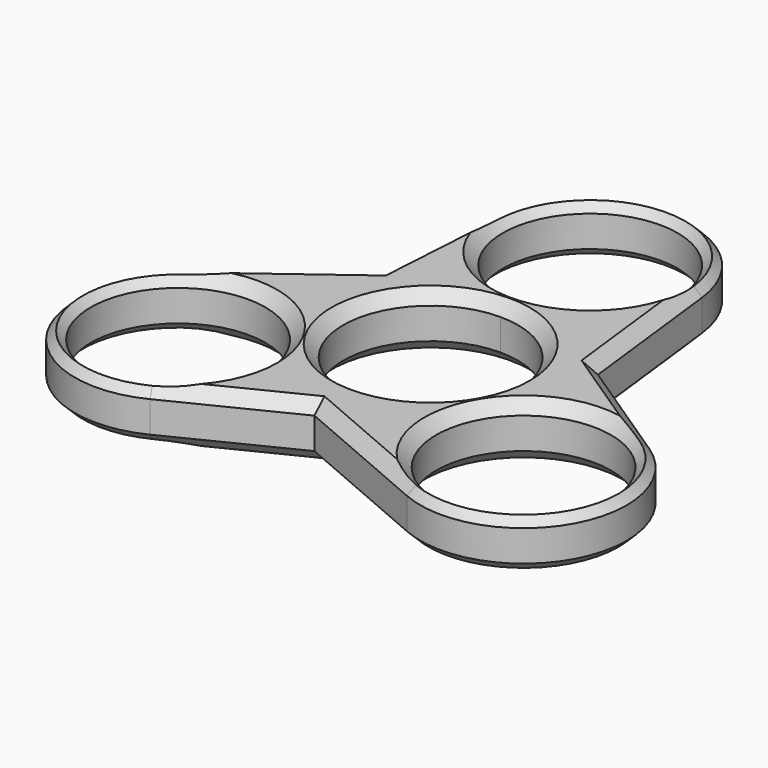
from build123d import *

# Parameters (mm, degrees)
F0_R         = 11.2
F1_DEPTH     = 7
F2_T4_DEPTH  = 23.5617897445
F2_T7_ANGLE  = 169.7193644143
F2_T11_DEPTH = 20.6774904565
F2_T16_DEPTH = 23.5617897445
F2_T19_ANGLE = 169.7193644143
F2_T23_DEPTH = 20.6774904565
F2_T28_DEPTH = 23.5617897445
F2_T31_ANGLE = 169.7193644143
F2_T35_DEPTH = 20.6774904565
F2_T49_DEPTH = 23.5617897445
F2_T53_DEPTH = 20.6774904565
F2_T60_DEPTH = 20.6774904565
F2_T64_DEPTH = 23.5617897445
F2_T71_DEPTH = 20.6774904565
F2_T75_DEPTH = 23.5617897445
F3_T4_DEPTH  = 23.5617897445
F3_T7_ANGLE  = 169.7193644143
F3_T11_DEPTH = 20.6774904565
F3_T16_DEPTH = 23.5617897445
F3_T19_ANGLE = 169.7193644143
F3_T23_DEPTH = 20.6774904565
F3_T28_DEPTH = 23.5617897445
F3_T31_ANGLE = 169.7193644143
F3_T35_DEPTH = 20.6774904565
F3_T49_DEPTH = 23.5617897445
F3_T53_DEPTH = 20.6774904565
F3_T60_DEPTH = 23.5617897445
F3_T64_DEPTH = 20.6774904565
F3_T71_DEPTH = 23.5617897445
F3_T75_DEPTH = 20.6774904565


# Not quite as in the source:
# - a fillet or chamfer that OpenCascade refuses, or shapes differently, is made with other operations: its cross-section is extruded or revolved along the edge and cut away or added


with BuildPart() as f1:
    # F0 (on Top) → F1 (new body)
    with BuildSketch(Plane.XY):
        with BuildLine():
            Line((15.4120276741, 7.5237850523), (13.109573538, 27.0930664517))
            ThreePointArc((13.109573538, 27.0930664517), (-0.3616695295, 38.7456835975), (-13.1743812219, 26.3726364702))
            Line((-13.1743812219, 26.3726364702), (-14.221802825, 9.5853149634))
            Line((-14.221802825, 9.5853149634), (-30.0180705826, -2.1933095092))
            ThreePointArc((-30.0180705826, -2.1933095092), (-33.3739115177, -19.686056799), (-16.252182537, -24.5956670524))
            Line((-16.252182537, -24.5956670524), (-1.1902248491, -17.1091000158))
            Line((-1.1902248491, -17.1091000158), (16.9084970446, -24.8997569426))
            ThreePointArc((16.9084970446, -24.8997569426), (33.7355810471, -19.0596267984), (29.4265637589, -1.7769694177))
            Line((29.4265637589, -1.7769694177), (15.4120276741, 7.5237850523))
        make_face()
        with Locations((-22.1275026794, -12.7753196284)):
            Circle(F0_R, mode=Mode.SUBTRACT)
        with Locations((22.1275026794, -12.7753196284)):
            Circle(F0_R, mode=Mode.SUBTRACT)
        with BuildLine():
            ThreePointArc((0, 11.2), (7.9195959493, 7.9195959493), (11.2, 0))
            ThreePointArc((11.2, 0), (5.6, -9.6994845224), (-5.6, -9.6994845224))
            ThreePointArc((-5.6, -9.6994845224), (-10.8183692544, 2.8987733051), (0, 11.2))
        make_face(mode=Mode.SUBTRACT)
        with Locations((0, 25.5506392568)):
            Circle(F0_R, mode=Mode.SUBTRACT)
    extrude(amount=F1_DEPTH)

    # F2: chamfer of 1.5 on 13 edges, made by hand


with BuildPart() as f2_tool2:
    # F2_s3 → F2_t4 (new body)
    with BuildSketch(Plane(origin=(-0.211945286, 1.8013896037, 0), x_dir=(0, 0, 1), z_dir=(-0.1168505451, 0.9931495105, 0))):
        Polygon((5.5, 16.185606124), (7, 14.685606124), (7, 16.185606124), align=None)
    extrude(amount=F2_T4_DEPTH)

    split(bisect_by=Plane(origin=(8.1788758548, 12.3240701783, 0), x_dir=(0, 0, 1), z_dir=(0.5529591727, 0.8332083493, 0)), keep=Keep.TOP)


with BuildPart() as f1_1:
    add(f1.part)

    # F2_t1: cut F2_tool2
    add(f2_tool2.part, mode=Mode.SUBTRACT)

    # F2_s6 → F2_t7 (revolve, cut)
    with BuildSketch(Plane(origin=(-2.9651532605, 25.2017695539, 0), x_dir=(0, 0, 1), z_dir=(0.1168505451, -0.9931495105, 0))):
        Polygon((7, -14.685606124), (5.5, -16.185606124), (7, -16.185606124), align=None)
    revolve(axis=Axis((0, 25.5506392568, 7), (0, 0, 1)), revolution_arc=F2_T7_ANGLE, mode=Mode.SUBTRACT)


with BuildPart() as f2_tool9:
    # F2_s10 → F2_t11 (new body)
    with BuildSketch(Plane(origin=(1.5880145579, 25.4515572947, 0), x_dir=(0, 0, 1), z_dir=(-0.0622725162, -0.9980591835, 0))):
        Polygon((7, 13.2911025961), (5.5, 14.7911025961), (7, 14.7911025961), align=None)
    extrude(amount=F2_T11_DEPTH)

    split(bisect_by=Plane(origin=(-9.6752745589, 12.9754733174, 0), x_dir=(0, 0, 1), z_dir=(-0.5977702957, 0.8016674333, 0)), keep=Keep.TOP)


with BuildPart() as f1_2:
    add(f1_1.part)

    # F2_t8: cut F2_tool9
    add(f2_tool9.part, mode=Mode.SUBTRACT)


with BuildPart() as f2_tool14:
    # F2_s15 → F2_t16 (new body)
    with BuildSketch(Plane(origin=(-1.4540765159, -1.0842448037, 0), x_dir=(0, 0, 1), z_dir=(-0.8016674333, -0.5977702957, 0))):
        Polygon((7, 14.685606124), (5.5, 16.185606124), (7, 16.185606124), align=None)
    extrude(amount=F2_T16_DEPTH)

    split(bisect_by=Plane(origin=(-14.7623957799, 0.9210791755, 0), x_dir=(0, 0, 1), z_dir=(-0.9980591835, 0.0622725162, 0)), keep=Keep.TOP)


with BuildPart() as f1_3:
    add(f1_2.part)

    # F2_t13: cut F2_tool14
    add(f2_tool14.part, mode=Mode.SUBTRACT)

    # F2_s18 → F2_t19 (revolve, cut)
    with BuildSketch(Plane(origin=(-20.3427960238, -15.1687828266, 0), x_dir=(0, 0, 1), z_dir=(0.8016674333, 0.5977702957, 0))):
        Polygon((7, -14.685606124), (5.5, -16.185606124), (7, -16.185606124), align=None)
    revolve(axis=Axis((-22.1275026794, -12.7753196284, 7), (0, 0, 1)), revolution_arc=F2_T19_ANGLE, mode=Mode.SUBTRACT)


with BuildPart() as f2_tool21:
    # F2_s22 → F2_t23 (new body)
    with BuildSketch(Plane(origin=(-22.835702462, -11.3505176986, 0), x_dir=(0, 0, 1), z_dir=(0.8954808655, 0.4451000108, 0))):
        Polygon((7, 13.2911025961), (5.5, 14.7911025961), (7, 14.7911025961), align=None)
    extrude(amount=F2_T23_DEPTH)

    split(bisect_by=Plane(origin=(-6.3994522396, -14.8667702153, 0), x_dir=(0, 0, 1), z_dir=(-0.3953792148, -0.9185179783, 0)), keep=Keep.TOP)


with BuildPart() as f1_4:
    add(f1_3.part)

    # F2_t20: cut F2_tool21
    add(f2_tool21.part, mode=Mode.SUBTRACT)


with BuildPart() as f2_tool26:
    # F2_s27 → F2_t28 (new body)
    with BuildSketch(Plane(origin=(1.6660218019, -0.7171447999, 0), x_dir=(0, 0, 1), z_dir=(0.9185179783, -0.3953792148, 0))):
        Polygon((7, 14.685606124), (5.5, 16.185606124), (7, 16.185606124), align=None)
    extrude(amount=F2_T28_DEPTH)

    split(bisect_by=Plane(origin=(6.5835199251, -13.2451493538, 0), x_dir=(0, 0, 1), z_dir=(0.4451000108, -0.8954808655, 0)), keep=Keep.TOP)


with BuildPart() as f1_5:
    add(f1_4.part)

    # F2_t25: cut F2_tool26
    add(f2_tool26.part, mode=Mode.SUBTRACT)

    # F2_s30 → F2_t31 (revolve, cut)
    with BuildSketch(Plane(origin=(23.3079492842, -10.0329867273, 0), x_dir=(0, 0, 1), z_dir=(-0.9185179783, 0.3953792148, 0))):
        Polygon((7, -14.685606124), (5.5, -16.185606124), (7, -16.185606124), align=None)
    revolve(axis=Axis((22.1275026794, -12.7753196284, 7), (0, 0, 1)), revolution_arc=F2_T31_ANGLE, mode=Mode.SUBTRACT)


with BuildPart() as f2_tool33:
    # F2_s34 → F2_t35 (new body)
    with BuildSketch(Plane(origin=(21.2476879041, -14.1010395961, 0), x_dir=(0, 0, 1), z_dir=(-0.8332083493, 0.5529591727, 0))):
        Polygon((7, 13.2911025961), (5.5, 14.7911025961), (7, 14.7911025961), align=None)
    extrude(amount=F2_T35_DEPTH)

    split(bisect_by=Plane(origin=(16.0747267985, 1.8912968978, 0), x_dir=(0, 0, 1), z_dir=(0.9931495105, 0.1168505451, 0)), keep=Keep.TOP)


with BuildPart() as f1_6:
    add(f1_5.part)

    # F2_t32: cut F2_tool33
    add(f2_tool33.part, mode=Mode.SUBTRACT)

    # F2_s37 → F2_t38 (revolve, cut)
    with BuildSketch(Plane.XZ.offset(12.7753196284)):
        Polygon((-9.4275026794, 7), (-10.9275026794, 5.5), (-10.9275026794, 7), align=None)
    revolve(axis=Axis((-22.1275026794, -12.7753196284, 7), (0, 0, 1)), mode=Mode.SUBTRACT)

    # F2_s39 → F2_t40 (revolve, cut)
    with BuildSketch(Plane.XZ.offset(12.7753196284)):
        Polygon((34.8275026794, 7), (33.3275026794, 5.5), (33.3275026794, 7), align=None)
    revolve(axis=Axis((22.1275026794, -12.7753196284, 7), (0, 0, 1)), mode=Mode.SUBTRACT)

    # F2_s41 → F2_t42 (revolve, cut)
    with BuildSketch(Plane(origin=(0, 0, 0), x_dir=(0, 0, 1), z_dir=(-0.8660254038, 0.5, 0))):
        Polygon((7, -12.7), (5.5, -11.2), (7, -11.2), align=None)
    revolve(axis=Axis((0, 0, 7), (0, 0, 1)), mode=Mode.SUBTRACT)

    # F2_s43 → F2_t44 (revolve, cut)
    with BuildSketch(Plane.XZ.offset(-25.5506392568)):
        Polygon((12.7, 7), (11.2, 5.5), (11.2, 7), align=None)
    revolve(axis=Axis((0, 25.5506392568, 7), (0, 0, 1)), mode=Mode.SUBTRACT)


with BuildPart() as f2_tool47:
    # F2_s48 → F2_t49 (new body)
    with BuildSketch(Plane(origin=(-0.211945286, 1.8013896037, 0), x_dir=(0, 0, 1), z_dir=(-0.1168505451, 0.9931495105, 0))):
        Polygon((5.5, 16.185606124), (7, 14.685606124), (7, 16.185606124), align=None)
    extrude(amount=F2_T49_DEPTH)

    split(bisect_by=Plane(origin=(8.1788758548, 12.3240701783, 0), x_dir=(0, 0, 1), z_dir=(-0.5529591727, -0.8332083493, 0)), keep=Keep.TOP)


with BuildPart() as f2_tool51:
    # F2_s52 → F2_t53 (new body)
    with BuildSketch(Plane(origin=(21.2476879041, -14.1010395961, 0), x_dir=(0, 0, 1), z_dir=(-0.8332083493, 0.5529591727, 0))):
        Polygon((7, 13.2911025961), (5.5, 14.7911025961), (7, 14.7911025961), align=None)
    extrude(amount=F2_T53_DEPTH)

    split(bisect_by=Plane(origin=(16.0747267985, 1.8912968978, 0), x_dir=(0, 0, 1), z_dir=(-0.9931495105, -0.1168505451, 0)), keep=Keep.TOP)


with BuildPart() as f2_tool47_1:
    add(f2_tool47.part)

    # F2_t55: intersect F2_tool51
    add(f2_tool51.part, mode=Mode.INTERSECT)


with BuildPart() as f1_7:
    add(f1_6.part)

    # F2_t45: cut F2_tool47
    add(f2_tool47_1.part, mode=Mode.SUBTRACT)


with BuildPart() as f2_tool58:
    # F2_s59 → F2_t60 (new body)
    with BuildSketch(Plane(origin=(1.5880145579, 25.4515572947, 0), x_dir=(0, 0, 1), z_dir=(-0.0622725162, -0.9980591835, 0))):
        Polygon((7, 13.2911025961), (5.5, 14.7911025961), (7, 14.7911025961), align=None)
    extrude(amount=F2_T60_DEPTH)

    split(bisect_by=Plane(origin=(-9.6752745589, 12.9754733174, 0), x_dir=(0, 0, 1), z_dir=(0.5977702957, -0.8016674333, 0)), keep=Keep.TOP)


with BuildPart() as f2_tool62:
    # F2_s63 → F2_t64 (new body)
    with BuildSketch(Plane(origin=(-1.4540765159, -1.0842448037, 0), x_dir=(0, 0, 1), z_dir=(-0.8016674333, -0.5977702957, 0))):
        Polygon((7, 14.685606124), (5.5, 16.185606124), (7, 16.185606124), align=None)
    extrude(amount=F2_T64_DEPTH)

    split(bisect_by=Plane(origin=(-14.7623957799, 0.9210791755, 0), x_dir=(0, 0, 1), z_dir=(0.9980591835, -0.0622725162, 0)), keep=Keep.TOP)


with BuildPart() as f2_tool58_1:
    add(f2_tool58.part)

    # F2_t66: intersect F2_tool62
    add(f2_tool62.part, mode=Mode.INTERSECT)


with BuildPart() as f1_8:
    add(f1_7.part)

    # F2_t56: cut F2_tool58
    add(f2_tool58_1.part, mode=Mode.SUBTRACT)


with BuildPart() as f2_tool69:
    # F2_s70 → F2_t71 (new body)
    with BuildSketch(Plane(origin=(-22.835702462, -11.3505176986, 0), x_dir=(0, 0, 1), z_dir=(0.8954808655, 0.4451000108, 0))):
        Polygon((7, 13.2911025961), (5.5, 14.7911025961), (7, 14.7911025961), align=None)
    extrude(amount=F2_T71_DEPTH)

    split(bisect_by=Plane(origin=(-6.3994522396, -14.8667702153, 0), x_dir=(0, 0, 1), z_dir=(0.3953792148, 0.9185179783, 0)), keep=Keep.TOP)


with BuildPart() as f2_tool73:
    # F2_s74 → F2_t75 (new body)
    with BuildSketch(Plane(origin=(1.6660218019, -0.7171447999, 0), x_dir=(0, 0, 1), z_dir=(0.9185179783, -0.3953792148, 0))):
        Polygon((7, 14.685606124), (5.5, 16.185606124), (7, 16.185606124), align=None)
    extrude(amount=F2_T75_DEPTH)

    split(bisect_by=Plane(origin=(6.5835199251, -13.2451493538, 0), x_dir=(0, 0, 1), z_dir=(-0.4451000108, 0.8954808655, 0)), keep=Keep.TOP)


with BuildPart() as f2_tool69_1:
    add(f2_tool69.part)

    # F2_t77: intersect F2_tool73
    add(f2_tool73.part, mode=Mode.INTERSECT)


with BuildPart() as f1_9:
    add(f1_8.part)

    # F2_t67: cut F2_tool69
    add(f2_tool69_1.part, mode=Mode.SUBTRACT)

    # F3: chamfer of 1.5 on 13 edges, made by hand


with BuildPart() as f3_tool2:
    # F3_s3 → F3_t4 (new body)
    with BuildSketch(Plane(origin=(-0.211945286, 1.8013896037, 0), x_dir=(0, 0, 1), z_dir=(-0.1168505451, 0.9931495105, 0))):
        Polygon((1.5, 16.185606124), (0, 14.685606124), (0, 16.185606124), align=None)
    extrude(amount=F3_T4_DEPTH)

    split(bisect_by=Plane(origin=(8.1788758548, 12.3240701783, 0), x_dir=(0, 0, 1), z_dir=(0.5529591727, 0.8332083493, 0)), keep=Keep.TOP)


with BuildPart() as f1_10:
    add(f1_9.part)

    # F3_t1: cut F3_tool2
    add(f3_tool2.part, mode=Mode.SUBTRACT)

    # F3_s6 → F3_t7 (revolve, cut)
    with BuildSketch(Plane(origin=(-2.9651532605, 25.2017695539, 0), x_dir=(0, 0, 1), z_dir=(0.1168505451, -0.9931495105, 0))):
        Polygon((1.5, -16.185606124), (0, -14.685606124), (0, -16.185606124), align=None)
    revolve(axis=Axis((0, 25.5506392568, 0), (0, 0, 1)), revolution_arc=F3_T7_ANGLE, mode=Mode.SUBTRACT)


with BuildPart() as f3_tool9:
    # F3_s10 → F3_t11 (new body)
    with BuildSketch(Plane(origin=(1.5880145579, 25.4515572947, 0), x_dir=(0, 0, 1), z_dir=(-0.0622725162, -0.9980591835, 0))):
        Polygon((1.5, 14.7911025961), (0, 13.2911025961), (0, 14.7911025961), align=None)
    extrude(amount=F3_T11_DEPTH)

    split(bisect_by=Plane(origin=(-9.6752745589, 12.9754733174, 0), x_dir=(0, 0, 1), z_dir=(-0.5977702957, 0.8016674333, 0)), keep=Keep.TOP)


with BuildPart() as f1_11:
    add(f1_10.part)

    # F3_t8: cut F3_tool9
    add(f3_tool9.part, mode=Mode.SUBTRACT)


with BuildPart() as f3_tool14:
    # F3_s15 → F3_t16 (new body)
    with BuildSketch(Plane(origin=(-1.4540765159, -1.0842448037, 0), x_dir=(0, 0, 1), z_dir=(-0.8016674333, -0.5977702957, 0))):
        Polygon((1.5, 16.185606124), (0, 14.685606124), (0, 16.185606124), align=None)
    extrude(amount=F3_T16_DEPTH)

    split(bisect_by=Plane(origin=(-14.7623957799, 0.9210791755, 0), x_dir=(0, 0, 1), z_dir=(-0.9980591835, 0.0622725162, 0)), keep=Keep.TOP)


with BuildPart() as f1_12:
    add(f1_11.part)

    # F3_t13: cut F3_tool14
    add(f3_tool14.part, mode=Mode.SUBTRACT)

    # F3_s18 → F3_t19 (revolve, cut)
    with BuildSketch(Plane(origin=(-20.3427960238, -15.1687828266, 0), x_dir=(0, 0, 1), z_dir=(0.8016674333, 0.5977702957, 0))):
        Polygon((1.5, -16.185606124), (0, -14.685606124), (0, -16.185606124), align=None)
    revolve(axis=Axis((-22.1275026794, -12.7753196284, 0), (0, 0, 1)), revolution_arc=F3_T19_ANGLE, mode=Mode.SUBTRACT)


with BuildPart() as f3_tool21:
    # F3_s22 → F3_t23 (new body)
    with BuildSketch(Plane(origin=(-22.835702462, -11.3505176986, 0), x_dir=(0, 0, 1), z_dir=(0.8954808655, 0.4451000108, 0))):
        Polygon((1.5, 14.7911025961), (0, 13.2911025961), (0, 14.7911025961), align=None)
    extrude(amount=F3_T23_DEPTH)

    split(bisect_by=Plane(origin=(-6.3994522396, -14.8667702153, 0), x_dir=(0, 0, 1), z_dir=(-0.3953792148, -0.9185179783, 0)), keep=Keep.TOP)


with BuildPart() as f1_13:
    add(f1_12.part)

    # F3_t20: cut F3_tool21
    add(f3_tool21.part, mode=Mode.SUBTRACT)


with BuildPart() as f3_tool26:
    # F3_s27 → F3_t28 (new body)
    with BuildSketch(Plane(origin=(1.6660218019, -0.7171447999, 0), x_dir=(0, 0, 1), z_dir=(0.9185179783, -0.3953792148, 0))):
        Polygon((1.5, 16.185606124), (0, 14.685606124), (0, 16.185606124), align=None)
    extrude(amount=F3_T28_DEPTH)

    split(bisect_by=Plane(origin=(6.5835199251, -13.2451493538, 0), x_dir=(0, 0, 1), z_dir=(0.4451000108, -0.8954808655, 0)), keep=Keep.TOP)


with BuildPart() as f1_14:
    add(f1_13.part)

    # F3_t25: cut F3_tool26
    add(f3_tool26.part, mode=Mode.SUBTRACT)

    # F3_s30 → F3_t31 (revolve, cut)
    with BuildSketch(Plane(origin=(23.3079492842, -10.0329867273, 0), x_dir=(0, 0, 1), z_dir=(-0.9185179783, 0.3953792148, 0))):
        Polygon((1.5, -16.185606124), (0, -14.685606124), (0, -16.185606124), align=None)
    revolve(axis=Axis((22.1275026794, -12.7753196284, 0), (0, 0, 1)), revolution_arc=F3_T31_ANGLE, mode=Mode.SUBTRACT)


with BuildPart() as f3_tool33:
    # F3_s34 → F3_t35 (new body)
    with BuildSketch(Plane(origin=(21.2476879041, -14.1010395961, 0), x_dir=(0, 0, 1), z_dir=(-0.8332083493, 0.5529591727, 0))):
        Polygon((1.5, 14.7911025961), (0, 13.2911025961), (0, 14.7911025961), align=None)
    extrude(amount=F3_T35_DEPTH)

    split(bisect_by=Plane(origin=(16.0747267985, 1.8912968978, 0), x_dir=(0, 0, 1), z_dir=(0.9931495105, 0.1168505451, 0)), keep=Keep.TOP)


with BuildPart() as f1_15:
    add(f1_14.part)

    # F3_t32: cut F3_tool33
    add(f3_tool33.part, mode=Mode.SUBTRACT)

    # F3_s37 → F3_t38 (revolve, cut)
    with BuildSketch(Plane.XZ.offset(12.7753196284)):
        Polygon((-10.9275026794, 1.5), (-9.4275026794, 0), (-10.9275026794, 0), align=None)
    revolve(axis=Axis((-22.1275026794, -12.7753196284, 0), (0, 0, 1)), mode=Mode.SUBTRACT)

    # F3_s39 → F3_t40 (revolve, cut)
    with BuildSketch(Plane.XZ.offset(12.7753196284)):
        Polygon((33.3275026794, 1.5), (34.8275026794, 0), (33.3275026794, 0), align=None)
    revolve(axis=Axis((22.1275026794, -12.7753196284, 0), (0, 0, 1)), mode=Mode.SUBTRACT)

    # F3_s41 → F3_t42 (revolve, cut)
    with BuildSketch(Plane(origin=(0, 0, 0), x_dir=(0, 0, 1), z_dir=(0.8660254038, -0.5, 0))):
        Polygon((1.5, 11.2), (0, 12.7), (0, 11.2), align=None)
    revolve(axis=Axis((0, 0, 0), (0, 0, -1)), mode=Mode.SUBTRACT)

    # F3_s43 → F3_t44 (revolve, cut)
    with BuildSketch(Plane.XZ.offset(-25.5506392568)):
        Polygon((11.2, 1.5), (12.7, 0), (11.2, 0), align=None)
    revolve(axis=Axis((0, 25.5506392568, 0), (0, 0, 1)), mode=Mode.SUBTRACT)


with BuildPart() as f3_tool47:
    # F3_s48 → F3_t49 (new body)
    with BuildSketch(Plane(origin=(-0.211945286, 1.8013896037, 0), x_dir=(0, 0, 1), z_dir=(-0.1168505451, 0.9931495105, 0))):
        Polygon((1.5, 16.185606124), (0, 14.685606124), (0, 16.185606124), align=None)
    extrude(amount=F3_T49_DEPTH)

    split(bisect_by=Plane(origin=(8.1788758548, 12.3240701783, 0), x_dir=(0, 0, 1), z_dir=(-0.5529591727, -0.8332083493, 0)), keep=Keep.TOP)


with BuildPart() as f3_tool51:
    # F3_s52 → F3_t53 (new body)
    with BuildSketch(Plane(origin=(21.2476879041, -14.1010395961, 0), x_dir=(0, 0, 1), z_dir=(-0.8332083493, 0.5529591727, 0))):
        Polygon((1.5, 14.7911025961), (0, 13.2911025961), (0, 14.7911025961), align=None)
    extrude(amount=F3_T53_DEPTH)

    split(bisect_by=Plane(origin=(16.0747267985, 1.8912968978, 0), x_dir=(0, 0, 1), z_dir=(-0.9931495105, -0.1168505451, 0)), keep=Keep.TOP)


with BuildPart() as f3_tool47_1:
    add(f3_tool47.part)

    # F3_t55: intersect F3_tool51
    add(f3_tool51.part, mode=Mode.INTERSECT)


with BuildPart() as f1_16:
    add(f1_15.part)

    # F3_t45: cut F3_tool47
    add(f3_tool47_1.part, mode=Mode.SUBTRACT)


with BuildPart() as f3_tool58:
    # F3_s59 → F3_t60 (new body)
    with BuildSketch(Plane(origin=(-1.4540765159, -1.0842448037, 0), x_dir=(0, 0, 1), z_dir=(-0.8016674333, -0.5977702957, 0))):
        Polygon((1.5, 16.185606124), (0, 14.685606124), (0, 16.185606124), align=None)
    extrude(amount=F3_T60_DEPTH)

    split(bisect_by=Plane(origin=(-14.7623957799, 0.9210791755, 0), x_dir=(0, 0, 1), z_dir=(0.9980591835, -0.0622725162, 0)), keep=Keep.TOP)


with BuildPart() as f3_tool62:
    # F3_s63 → F3_t64 (new body)
    with BuildSketch(Plane(origin=(1.5880145579, 25.4515572947, 0), x_dir=(0, 0, 1), z_dir=(-0.0622725162, -0.9980591835, 0))):
        Polygon((1.5, 14.7911025961), (0, 13.2911025961), (0, 14.7911025961), align=None)
    extrude(amount=F3_T64_DEPTH)

    split(bisect_by=Plane(origin=(-9.6752745589, 12.9754733174, 0), x_dir=(0, 0, 1), z_dir=(0.5977702957, -0.8016674333, 0)), keep=Keep.TOP)


with BuildPart() as f3_tool58_1:
    add(f3_tool58.part)

    # F3_t66: intersect F3_tool62
    add(f3_tool62.part, mode=Mode.INTERSECT)


with BuildPart() as f1_17:
    add(f1_16.part)

    # F3_t56: cut F3_tool58
    add(f3_tool58_1.part, mode=Mode.SUBTRACT)


with BuildPart() as f3_tool69:
    # F3_s70 → F3_t71 (new body)
    with BuildSketch(Plane(origin=(1.6660218019, -0.7171447999, 0), x_dir=(0, 0, 1), z_dir=(0.9185179783, -0.3953792148, 0))):
        Polygon((1.5, 16.185606124), (0, 14.685606124), (0, 16.185606124), align=None)
    extrude(amount=F3_T71_DEPTH)

    split(bisect_by=Plane(origin=(6.5835199251, -13.2451493538, 0), x_dir=(0, 0, 1), z_dir=(-0.4451000108, 0.8954808655, 0)), keep=Keep.TOP)


with BuildPart() as f3_tool73:
    # F3_s74 → F3_t75 (new body)
    with BuildSketch(Plane(origin=(-22.835702462, -11.3505176986, 0), x_dir=(0, 0, 1), z_dir=(0.8954808655, 0.4451000108, 0))):
        Polygon((1.5, 14.7911025961), (0, 13.2911025961), (0, 14.7911025961), align=None)
    extrude(amount=F3_T75_DEPTH)

    split(bisect_by=Plane(origin=(-6.3994522396, -14.8667702153, 0), x_dir=(0, 0, 1), z_dir=(0.3953792148, 0.9185179783, 0)), keep=Keep.TOP)


with BuildPart() as f3_tool69_1:
    add(f3_tool69.part)

    # F3_t77: intersect F3_tool73
    add(f3_tool73.part, mode=Mode.INTERSECT)


with BuildPart() as f1_18:
    add(f1_17.part)

    # F3_t67: cut F3_tool69
    add(f3_tool69_1.part, mode=Mode.SUBTRACT)


solid = f1_18.part
